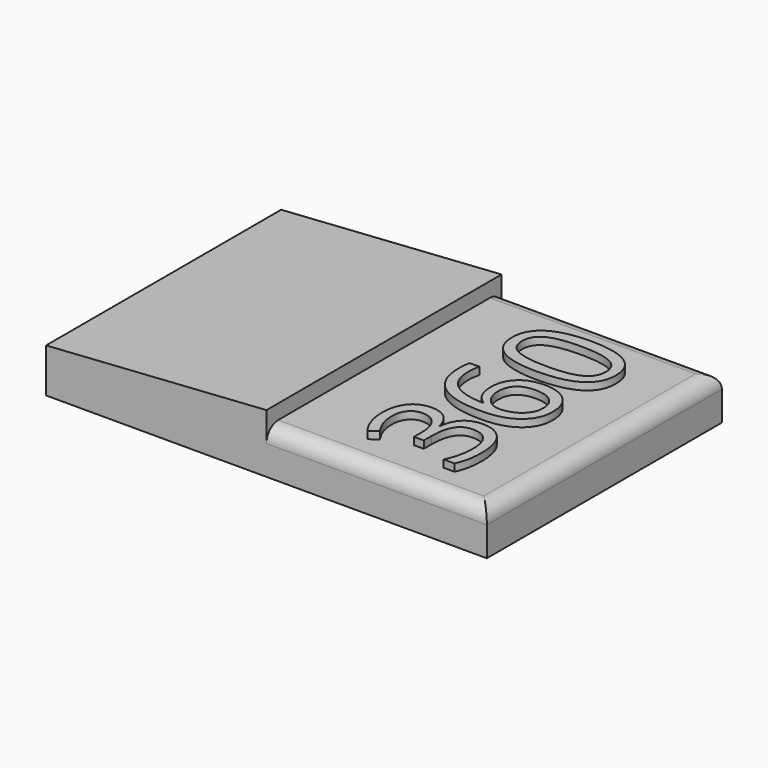
from build123d import *

# Parameters (mm, degrees)
F1_DEPTH     = 20
F2_TEXT_SIZE = 9.5848436295
F3_DEPTH     = 0.5
F4_R         = 1


# Not quite as in the source:
# - Text() gives the source's letters only with a copy of the font that has no kerning and outlines rounded to 1/6400 em; it was checked with that copy


with BuildPart() as f1:
    # F0 (on Front) → F1 (new body)
    with BuildSketch(Plane.XZ):
        Polygon((0, 3), (0, 0), (30, 0), (30, 3), (15, 3), (15, 4), align=None)
    extrude(amount=F1_DEPTH)

    # F2 (on face) → F3 (join)
    with BuildSketch(Plane.XY.offset(3)):
        with Locations(Location((26.3114674158, -18.2382208109), (0, 0, 90))):
            Text('360', F2_TEXT_SIZE, font='Open Sans', text_align=(TextAlign.LEFT, TextAlign.BOTTOM))
    extrude(amount=F3_DEPTH)

    # F4
    f4_edges = [f1.edges().sort_by_distance(p)[0] for p in [
        (22.5, -20, 3),
        (30, -10, 3),
        (22.5, 0, 3),
    ]]
    fillet(f4_edges, radius=F4_R)


solid = f1.part
